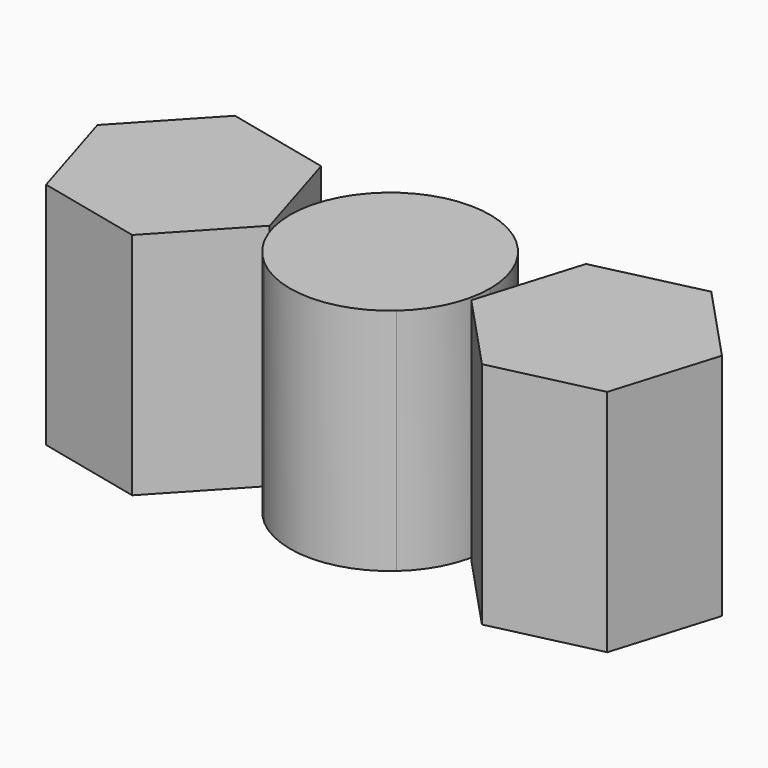
from build123d import *

# Parameters (mm, degrees)
F1_DEPTH = 25


# Not quite as in the source:
# - a feature of the source that left no trace in its solid (it failed there, or was rolled back) is left out


with BuildPart() as f1:
    # F0 (on Top) → F1 (new body)
    with BuildSketch(Plane.XY):
        Polygon((-10.9947116086, -2.6709130821), (-14.4468207234, 8.6501414622), (-25.9771961137, 11.3210545442), (-34.0554623892, 2.6709130821), (-30.6033532745, -8.6501414622), (-19.0729778841, -11.3210545442), align=None)
    extrude(amount=F1_DEPTH)


with BuildPart() as f1b:
    # F0 (on Top) → F1, piece 2 (new body)
    with BuildSketch(Plane.XY):
        Polygon((25.9771961137, 11.3210545442), (14.4468207234, 8.6501414622), (10.9947116086, -2.6709130821), (19.0729778841, -11.3210545442), (30.6033532745, -8.6501414622), (34.0554623892, 2.6709130821), align=None)
    extrude(amount=F1_DEPTH)


with BuildPart() as f1c:
    # F0 (on Top) → F1, piece 3 (new body)
    with BuildSketch(Plane.XY):
        with BuildLine():
            ThreePointArc((7.2121566552, -8.1728083534), (9.9353537315, -4.4831625254), (10.9, 0))
            ThreePointArc((10.9, 0), (10.1984296374, 3.847341021), (8.1840306547, 7.1994195768))
            ThreePointArc((8.1840306547, 7.1994195768), (0.0683052099, 10.8997859795), (-8.0931588609, 7.3014231252))
            ThreePointArc((-8.0931588609, 7.3014231252), (-10.8759119881, -0.724250251), (-7.0535557785, -8.3100752632))
            ThreePointArc((-7.0535557785, -8.3100752632), (0.104876645, -10.899495442), (7.2121566552, -8.1728083534))
        make_face()
    extrude(amount=F1_DEPTH)


solid = Compound([f1.part, f1b.part, f1c.part])
